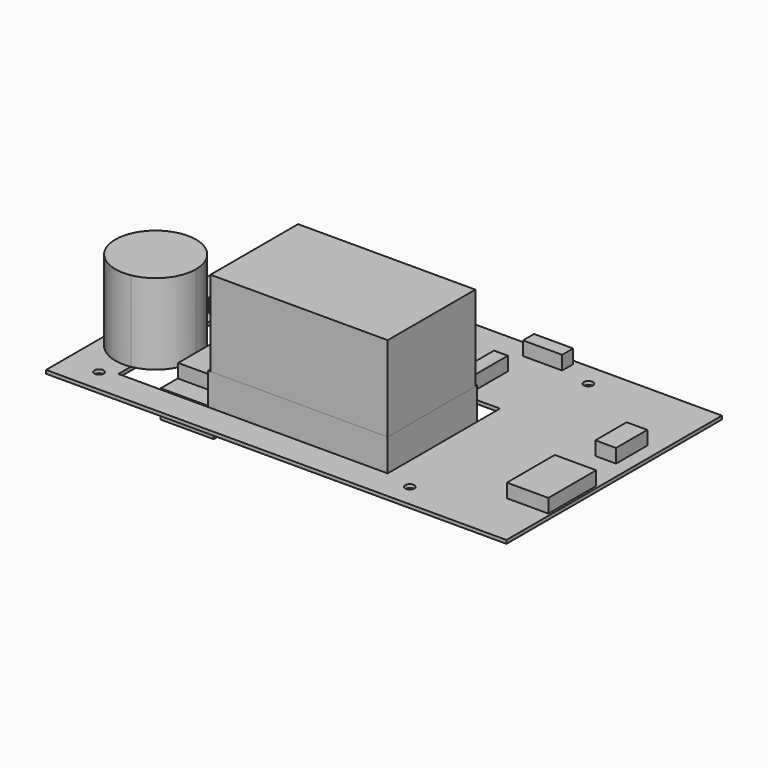
from build123d import *

# Parameters (mm, degrees)
F0_W      = 200
F0_H      = 117
F0_R      = 2
F0_W_2    = 117
F0_H_2    = 61
F1_DEPTH  = 1.5
F2_W      = 23
F2_H      = 7
F3_DEPTH  = 6
F2_W_2    = 17
F2_H_2    = 6
F2_W_3    = 6
F2_H_3    = 22
F2_W_4    = 18
F2_H_4    = 26
F2_H_5    = 27
F2_W_5    = 9
F2_H_6    = 17
F2_H_7    = 10
F4_DEPTH  = 35
F5_W      = 78
F5_H      = 48.6
F6_DEPTH  = 13.95
F7_W      = 77
F7_H      = 47.6
F8_DEPTH  = 37
F9_W      = 23
F9_H      = 11
F10_DEPTH = 12


with BuildPart() as f1:
    # F0 (on Top) → F1 (new body)
    with BuildSketch(Plane.XY):
        with Locations((11.1932437867, -14.8287359455)):
            Rectangle(F0_W, F0_H)
        with Locations((-73.8067562133, -63.3287359455)):
            Circle(F0_R, mode=Mode.SUBTRACT)
        with Locations((-9.3067562133, -29.8287359455)):
            Rectangle(F0_W_2, F0_H_2, mode=Mode.SUBTRACT)
        with Locations((61.1932437867, -63.3287359455)):
            Circle(F0_R, mode=Mode.SUBTRACT)
        with Locations((-73.8067562133, 33.6712640545)):
            Circle(F0_R, mode=Mode.SUBTRACT)
        with Locations((61.1932437867, 33.6712640545)):
            Circle(F0_R, mode=Mode.SUBTRACT)
    extrude(amount=F1_DEPTH)


with BuildPart() as f3:
    # F2 (on face) → F3 (new body)
    with BuildSketch(Plane.XY.offset(1.5)):
        with Locations((-6.3067562133, 37.1712640545)):
            Rectangle(F2_W, F2_H)
    extrude(amount=F3_DEPTH)


with BuildPart() as f3b:
    # F2 (on face) → F3, piece 2 (new body)
    with BuildSketch(Plane.XY.offset(1.5)):
        with Locations((39.6932437867, 38.6712640545)):
            Rectangle(F2_W_2, F2_H_2)
    extrude(amount=F3_DEPTH)


with BuildPart() as f3c:
    # F2 (on face) → F3, piece 3 (new body)
    with BuildSketch(Plane.XY.offset(1.5)):
        with Locations((31.1932437867, 12.6712640545)):
            Rectangle(F2_W_3, F2_H_3)
    extrude(amount=F3_DEPTH)


with BuildPart() as f3d:
    # F2 (on face) → F3, piece 4 (new body)
    with BuildSketch(Plane.XY.offset(1.5)):
        with Locations((101.1932437867, -36.3287359455)):
            Rectangle(F2_W_4, F2_H_4)
    extrude(amount=F3_DEPTH)


with BuildPart() as f3e:
    # F2 (on face) → F3, piece 5 (new body)
    with BuildSketch(Plane.XY.offset(1.5)):
        with Locations((-41.3067562133, -36.8287359455)):
            Rectangle(F2_W_2, F2_H_5)
    extrude(amount=F3_DEPTH)


with BuildPart() as f3f:
    # F2 (on face) → F3, piece 6 (new body)
    with BuildSketch(Plane.XY.offset(1.5)):
        Polygon((-71.8067562133, -6.3287359455), (-67.8067562133, -6.3287359455), (-67.8067562133, 0.6712640545), (-62.8067562133, 0.6712640545), (-62.8067562133, 15.6712640545), (-71.8067562133, 15.6712640545), align=None)
    extrude(amount=F3_DEPTH)


with BuildPart() as f3g:
    # F2 (on face) → F3, piece 7 (new body)
    with BuildSketch(Plane.XY.offset(1.5)):
        with Locations((100.6932437867, 2.1712640545)):
            Rectangle(F2_W_5, F2_H_6)
    extrude(amount=F3_DEPTH)


with BuildPart() as f3h:
    # F2 (on face) → F3, piece 8 (new body)
    with BuildSketch(Plane.XY.offset(1.5)):
        with Locations((-43.8067562133, 5.6712640545)):
            Rectangle(F2_W_3, F2_H_7)
    extrude(amount=F3_DEPTH)


with BuildPart() as f4:
    # F2 (on face) → F4 (new body)
    with BuildSketch(Plane.XY.offset(1.5)):
        with BuildLine():
            Line((-67.8067562133, -53.5696755951), (-67.8067562133, -19.087796296))
            ThreePointArc((-67.8067562133, -19.087796296), (-88.3067562133, -36.3287359455), (-67.8067562133, -53.5696755951))
        make_face()
        with BuildLine():
            ThreePointArc((-67.8067562133, -53.5696755951), (-57.4136609773, -47.5926162716), (-53.3067562133, -36.3287359455))
            ThreePointArc((-53.3067562133, -36.3287359455), (-57.4136609773, -25.0648556195), (-67.8067562133, -19.087796296))
            Line((-67.8067562133, -19.087796296), (-67.8067562133, -53.5696755951))
        make_face()
    extrude(amount=F4_DEPTH)


with BuildPart() as f6:
    # F5 (on face) → F6 (new body)
    with BuildSketch(Plane.XY.offset(1.5)):
        with Locations((10.1932437867, -36.0287359455)):
            Rectangle(F5_W, F5_H)
    extrude(amount=F6_DEPTH)


with BuildPart() as f8:
    # F7 (on face) → F8 (new body)
    with BuildSketch(Plane.XY.offset(15.45)):
        with Locations((10.6932437867, -36.5287359455)):
            Rectangle(F7_W, F7_H)
    extrude(amount=F8_DEPTH)


with BuildPart() as f10:
    # F9 (on face) → F10 (new body)
    with BuildSketch(Plane(origin=(0, 0, 0), x_dir=(1, 0, 0), z_dir=(0, 0, -1))):
        with Locations((-40.3067562133, 51.8287359455)):
            Rectangle(F9_W, F9_H)
    extrude(amount=F10_DEPTH)


solid = Compound([f1.part, f3.part, f3b.part, f3c.part, f3d.part, f3e.part, f3f.part, f3g.part, f3h.part, f4.part, f6.part, f8.part, f10.part])
